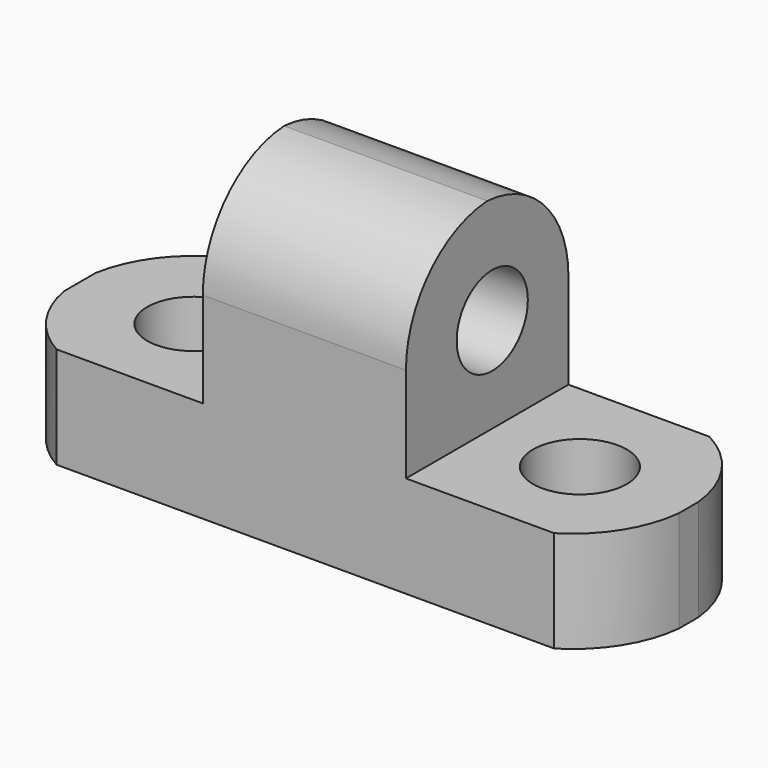
from build123d import *

# Parameters (mm, degrees)
F1_DEPTH    = 25.4
F3_DEPTH    = 25.4
F5_DEPTH    = 25.4
F6_T1_DEPTH = 92.8531269327
F7_R        = 5.5593746135
F8_DEPTH    = 25.4
F9_R        = 5.8665873172
F10_DEPTH   = 25.4
F9_R_2      = 5.7482740473
F11_DEPTH   = 25.4


# Not quite as in the source:
# - a fillet or chamfer that OpenCascade refuses, or shapes differently, is made with other operations: its cross-section is extruded or revolved along the edge and cut away or added


with BuildPart() as f1:
    # F0 (on Front) → F1 (new body)
    with BuildSketch(Plane.XZ):
        Polygon((25.4, 12.7), (0, 12.7), (0, 0), (76.2, 0), (76.2, 12.7), (50.8, 12.7), (50.8, 38.1), (25.4, 38.1), align=None)
    extrude(amount=F1_DEPTH)

    # F2 (on face) → F3 (cut)
    with BuildSketch(Plane.XY.offset(12.7)):
        with BuildLine():
            ThreePointArc((0, -10.3920384811), (2.632385222, -4.2752682762), (7.7379127033, 0))
            Line((7.7379127033, 0), (0, 0))
            Line((0, 0), (0, -10.3920384811))
        make_face()
        with BuildLine():
            ThreePointArc((7.1188798174, -25.4), (2.4265465189, -21.1696188601), (0, -15.3364389071))
            Line((0, -15.3364389071), (0, -25.4))
            Line((0, -25.4), (7.1188798174, -25.4))
        make_face()
    extrude(amount=-F3_DEPTH, mode=Mode.SUBTRACT)

    # F4 (on face) → F5 (cut)
    with BuildSketch(Plane.XY.offset(12.7)):
        with BuildLine():
            ThreePointArc((68.4031397104, 0), (73.7378443896, -4.7264477616), (76.2, -11.4149582241))
            Line((76.2, -11.4149582241), (76.2, 0))
            Line((76.2, 0), (68.4031397104, 0))
        make_face()
        with BuildLine():
            ThreePointArc((76.2, -14.5105812124), (74.030690178, -20.7530692397), (69.3316906691, -25.4))
            Line((69.3316906691, -25.4), (76.2, -25.4))
            Line((76.2, -25.4), (76.2, -14.5105812124))
        make_face()
    extrude(amount=-F5_DEPTH, mode=Mode.SUBTRACT)

    # F6: fillet of radius 13.4906253865 on 2 edges, made by hand

    # F6_s2 → F6_t1 (cut)
    with BuildSketch(Plane.YZ.offset(-8.3265634664)):
        with BuildLine():
            ThreePointArc((-25.4, 24.6093746135), (-21.4486873067, 34.1486873067), (-11.9093746135, 38.1))
            Line((-11.9093746135, 38.1), (-25.4, 38.1))
            Line((-25.4, 38.1), (-25.4, 24.6093746135))
        make_face()
        with BuildLine():
            ThreePointArc((0, 24.6093746135), (-3.9513126933, 34.1486873067), (-13.4906253865, 38.1))
            Line((-13.4906253865, 38.1), (0, 38.1))
            Line((0, 38.1), (0, 24.6093746135))
        make_face()
    extrude(amount=F6_T1_DEPTH, mode=Mode.SUBTRACT)

    # F7 (on face) → F8 (cut)
    with BuildSketch(Plane.YZ.offset(50.8)):
        with Locations((-11.9093746135, 24.6093746135)):
            Circle(F7_R)
    extrude(amount=-F8_DEPTH, mode=Mode.SUBTRACT)

    # F9 (on face) → F10 (cut)
    with BuildSketch(Plane.XY.offset(12.7)):
        with Locations((62.5223219395, -12.8642386941)):
            Circle(F9_R)
    extrude(amount=-F10_DEPTH, mode=Mode.SUBTRACT)

    # F9 (on face) → F11 (cut)
    with BuildSketch(Plane.XY.offset(12.7)):
        with Locations((14.1673966027, -12.8642386941)):
            Circle(F9_R_2)
    extrude(amount=-F11_DEPTH, mode=Mode.SUBTRACT)


solid = f1.part
